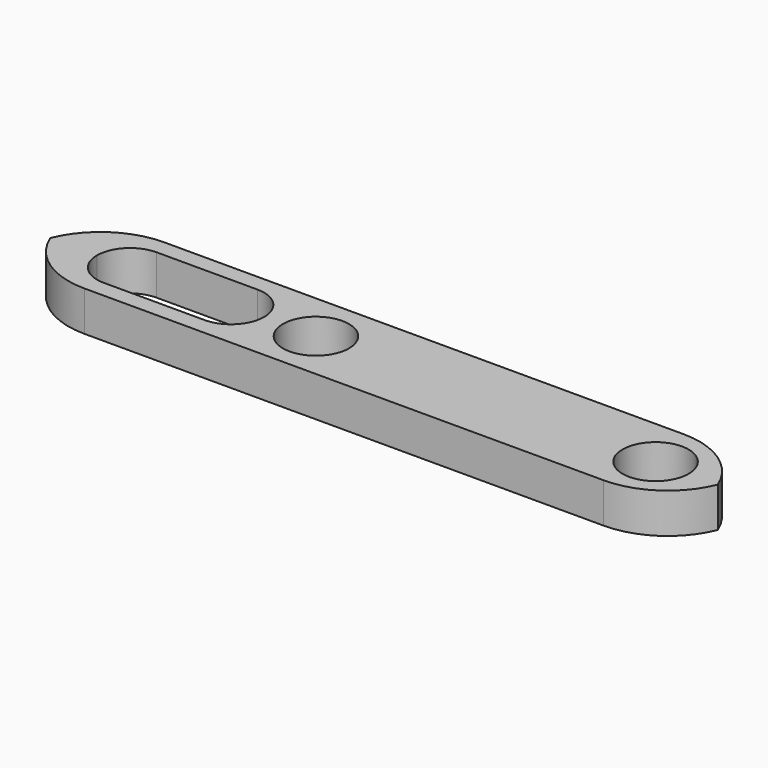
from build123d import *

# Parameters (mm, degrees)
F0_W        = 43.18
F0_H        = 6.35
F1_DEPTH    = 2.54
F2_T1_DEPTH = 27.94
F4_DEPTH    = 2.541


# Not quite as in the source:
# - a fillet or chamfer that OpenCascade refuses, or shapes differently, is made with other operations: its cross-section is extruded or revolved along the edge and cut away or added


with BuildPart() as f1:
    # F0 (on Top) → F1 (new body)
    with BuildSketch(Plane.XY):
        Rectangle(F0_W, F0_H)
    extrude(amount=F1_DEPTH)

    # F2: fillet of radius 5.08 on 4 edges, made by hand

    # F2_s2 → F2_t1 (cut)
    with BuildSketch(Plane.XY.offset(-12.7)):
        with BuildLine():
            ThreePointArc((21.59, 1.905), (20.1021024484, -1.6871024484), (16.51, -3.175))
            Line((16.51, -3.175), (21.59, -3.175))
            Line((21.59, -3.175), (21.59, 1.905))
        make_face()
        with BuildLine():
            ThreePointArc((21.59, -1.905), (20.1021024484, 1.6871024484), (16.51, 3.175))
            Line((16.51, 3.175), (21.59, 3.175))
            Line((21.59, 3.175), (21.59, -1.905))
        make_face()
        with BuildLine():
            ThreePointArc((-16.51, 3.175), (-20.1021024484, 1.6871024484), (-21.59, -1.905))
            Line((-21.59, -1.905), (-21.59, 3.175))
            Line((-21.59, 3.175), (-16.51, 3.175))
        make_face()
        with BuildLine():
            ThreePointArc((-21.59, 1.905), (-20.1021024484, -1.6871024484), (-16.51, -3.175))
            Line((-16.51, -3.175), (-21.59, -3.175))
            Line((-21.59, -3.175), (-21.59, 1.905))
        make_face()
    extrude(amount=F2_T1_DEPTH, mode=Mode.SUBTRACT)

    # F3 (on face) → F4 (cut, through all)
    with BuildSketch(Plane.XY.offset(2.54)):
        with BuildLine():
            Line((15.1645667607, 0), (19.3645667607, 0))
            ThreePointArc((19.3645667607, 0), (17.2645667607, 2.1), (15.1645667607, 0))
        make_face()
        with BuildLine():
            ThreePointArc((-9.7229412393, -2.1), (-8.2380169988, -1.4849242405), (-7.6229412393, 0))
            Line((-7.6229412393, 0), (-18.2392860393, 0))
            ThreePointArc((-18.2392860393, 0), (-17.6242102798, -1.4849242405), (-16.1392860393, -2.1))
            Line((-16.1392860393, -2.1), (-9.7229412393, -2.1))
        make_face()
        with BuildLine():
            Line((-18.2392860393, 0), (-7.6229412393, 0))
            ThreePointArc((-7.6229412393, 0), (-8.2380169988, 1.4849242405), (-9.7229412393, 2.1))
            Line((-9.7229412393, 2.1), (-16.1392860393, 2.1))
            ThreePointArc((-16.1392860393, 2.1), (-17.6242102798, 1.4849242405), (-18.2392860393, 0))
        make_face()
        with BuildLine():
            ThreePointArc((-6.4254332393, 0), (-4.3254332393, -2.1), (-2.2254332393, 0))
            Line((-2.2254332393, 0), (-6.4254332393, 0))
        make_face()
        with BuildLine():
            Line((-6.4254332393, 0), (-2.2254332393, 0))
            ThreePointArc((-2.2254332393, 0), (-4.3254332393, 2.1), (-6.4254332393, 0))
        make_face()
        with BuildLine():
            ThreePointArc((15.1645667607, 0), (17.2645667607, -2.1), (19.3645667607, 0))
            Line((19.3645667607, 0), (15.1645667607, 0))
        make_face()
    extrude(amount=-F4_DEPTH, mode=Mode.SUBTRACT)


solid = f1.part
